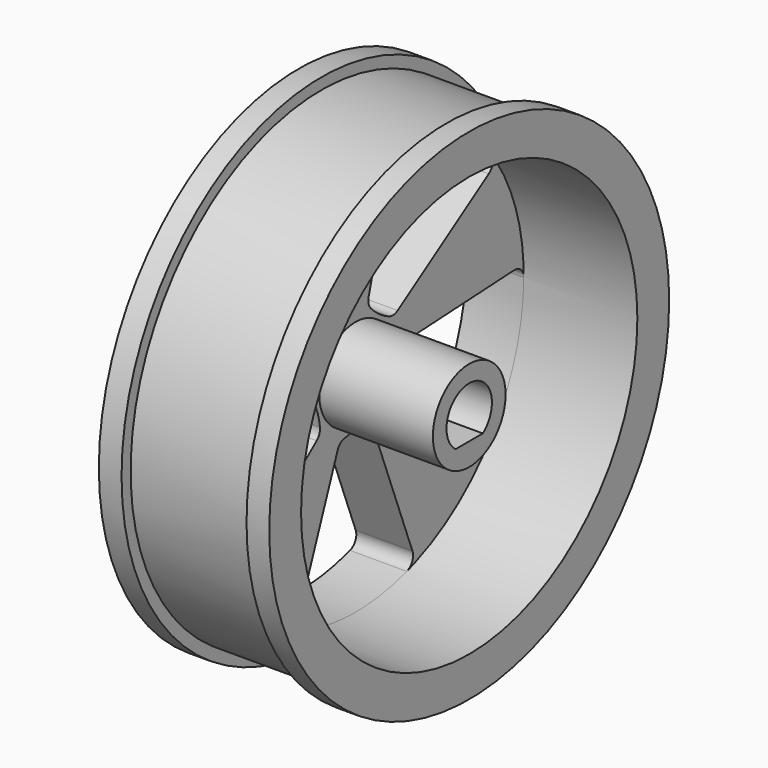
from build123d import *

# Parameters (mm, degrees)
F0_R         = 21
F1_DEPTH     = 5.5
F2_R         = 22
F3_DEPTH     = 2
F4_R         = 22
F5_DEPTH     = 2
F7_DEPTH     = 15.001
F8_R         = 18.5
F8_R_2       = 4
F9_DEPTH     = 10
F11_DEPTH    = 5.001
F12_T1_DEPTH = 5


# Not quite as in the source:
# - a fillet or chamfer that OpenCascade refuses, or shapes differently, is made with other operations: its cross-section is extruded or revolved along the edge and cut away or added


with BuildPart() as f1:
    # F0 (on Right) → F1 (new body, symmetric)
    with BuildSketch(Plane.YZ):
        Circle(F0_R)
    extrude(amount=F1_DEPTH, both=True)

    # F2 (on face) → F3 (join)
    with BuildSketch(Plane.YZ.offset(5.5)):
        Circle(F2_R)
    extrude(amount=F3_DEPTH)

    # F4 (on face) → F5 (join)
    with BuildSketch(Plane(origin=(-5.5, 0, 0), x_dir=(0, -1, 0), z_dir=(-1, 0, 0))):
        Circle(F4_R)
    extrude(amount=F5_DEPTH)

    # F6 (on face) → F7 (cut, through all)
    with BuildSketch(Plane(origin=(-7.5, 0, 0), x_dir=(0, -1, 0), z_dir=(-1, 0, 0))):
        with BuildLine():
            Line((-1.5, -2), (1.5, -2))
            ThreePointArc((1.5, -2), (0, 2.5), (-1.5, -2))
        make_face()
    extrude(amount=-F7_DEPTH, mode=Mode.SUBTRACT)

    # F8 (on face) → F9 (cut)
    with BuildSketch(Plane.YZ.offset(7.5)):
        Circle(F8_R)
        Circle(F8_R_2, mode=Mode.SUBTRACT)
    extrude(amount=-F9_DEPTH, mode=Mode.SUBTRACT)

    # F10 (on face) → F11 (cut, through all)
    with BuildSketch(Plane.YZ.offset(-2.5)):
        with BuildLine():
            Line((4.7881523344, 17.8696277863), (1.2940952255, 4.8296291314))
            ThreePointArc((1.2940952255, 4.8296291314), (2.5827855501, 3.5548993357), (4.1933528397, 2.7231951751))
            Line((4.1933528397, 2.7231951751), (15.515405507, 10.0758221478))
            ThreePointArc((15.515405507, 10.0758221478), (10.8740271674, 14.9668143959), (4.7881523344, 17.8696277863))
        make_face()
        with BuildLine():
            ThreePointArc((4.9931476738, 0.2616797812), (4.1790348058, -1.3578507196), (3.8857298073, -3.1466019552))
            Line((3.8857298073, -3.1466019552), (14.377200287, -11.6424272344))
            ThreePointArc((14.377200287, -11.6424272344), (17.5945455515, -5.7168143959), (18.474646393, 0.9682151905))
            Line((18.474646393, 0.9682151905), (4.9931476738, 0.2616797812))
        make_face()
        with BuildLine():
            ThreePointArc((1.7918397477, -4.6679021325), (0, -4.3940972321), (-1.7918397477, -4.6679021325))
            Line((-1.7918397477, -4.6679021325), (-6.6298070666, -17.2712378902))
            ThreePointArc((-6.6298070666, -17.2712378902), (0, -18.5), (6.6298070666, -17.2712378902))
            Line((6.6298070666, -17.2712378902), (1.7918397477, -4.6679021325))
        make_face()
        with BuildLine():
            ThreePointArc((-3.8857298073, -3.1466019552), (-4.1790348058, -1.3578507196), (-4.9931476738, 0.2616797812))
            Line((-4.9931476738, 0.2616797812), (-18.474646393, 0.9682151905))
            ThreePointArc((-18.474646393, 0.9682151905), (-17.5945455515, -5.7168143959), (-14.377200287, -11.6424272344))
            Line((-14.377200287, -11.6424272344), (-3.8857298073, -3.1466019552))
        make_face()
        with BuildLine():
            ThreePointArc((-4.1933528397, 2.7231951751), (-2.5827855501, 3.5548993357), (-1.2940952255, 4.8296291314))
            Line((-1.2940952255, 4.8296291314), (-4.7881523344, 17.8696277863))
            ThreePointArc((-4.7881523344, 17.8696277863), (-10.8740271674, 14.9668143959), (-15.515405507, 10.0758221478))
            Line((-15.515405507, 10.0758221478), (-4.1933528397, 2.7231951751))
        make_face()
    extrude(amount=-F11_DEPTH, mode=Mode.SUBTRACT)

    # F12: fillet of radius 1 on 20 edges, made by hand

    # F12_s2 → F12_t1 (join)
    with BuildSketch(Plane.YZ.offset(-7.5)):
        with BuildLine():
            ThreePointArc((4.6223226532, 3.0017714292), (4.1563467345, 2.8435407412), (3.671320929, 2.9267301361))
            ThreePointArc((3.671320929, 2.9267301361), (3.9299597122, 2.8188656209), (4.1933528397, 2.7231951751))
            Line((4.1933528397, 2.7231951751), (4.6223226532, 3.0017714292))
        make_face()
        with BuildLine():
            ThreePointArc((1.4264780248, 5.3236884645), (1.4199861758, 4.831623059), (1.6489852086, 4.3960430429))
            ThreePointArc((1.6489852086, 4.3960430429), (1.466476179, 4.6086911748), (1.2940952255, 4.8296291314))
            Line((1.2940952255, 4.8296291314), (1.4264780248, 5.3236884645))
        make_face()
        with BuildLine():
            ThreePointArc((14.65275333, 9.5156092737), (15.0918050058, 10.1744115971), (14.9142922547, 10.9459529755))
            ThreePointArc((14.9142922547, 10.9459529755), (15.221067912, 10.5151838604), (15.515405507, 10.0758221478))
            Line((15.515405507, 10.0758221478), (14.65275333, 9.5156092737))
        make_face()
        with BuildLine():
            ThreePointArc((4.521932413, 16.8760815136), (5.0128162263, 17.4972255847), (5.8014501386, 17.5668203238))
            ThreePointArc((5.8014501386, 17.5668203238), (5.2969654732, 17.7254663345), (4.7881523344, 17.8696277863))
            Line((4.7881523344, 17.8696277863), (4.521932413, 16.8760815136))
        make_face()
        with BuildLine():
            ThreePointArc((5.5039345567, 0.2884489874), (5.0339464546, 0.1425665301), (4.6904498348, -0.2098261196))
            ThreePointArc((4.6904498348, -0.2098261196), (4.8362918345, 0.0294621688), (4.9931476738, 0.2616797812))
            Line((4.9931476738, 0.2616797812), (5.5039345567, 0.2884489874))
        make_face()
        with BuildLine():
            ThreePointArc((4.2832305314, -3.4684916949), (3.9887497267, -3.0742182326), (3.9179863263, -2.5872243429))
            ThreePointArc((3.9179863263, -2.5872243429), (3.8953248556, -2.8665364113), (3.8857298073, -3.1466019552))
            Line((3.8857298073, -3.1466019552), (4.2832305314, -3.4684916949))
        make_face()
        with BuildLine():
            ThreePointArc((1.2498722119, -4.5257227166), (1.6911638308, -4.7435120977), (1.9751406031, -5.1454171863))
            Line((1.9751406031, -5.1454171863), (1.7918397477, -4.6679021325))
            ThreePointArc((1.7918397477, -4.6679021325), (1.5225165542, -4.5904825531), (1.2498722119, -4.5257227166))
        make_face()
        with BuildLine():
            ThreePointArc((-1.9751406031, -5.1454171863), (-1.6911638308, -4.7435120977), (-1.2498722119, -4.5257227166))
            ThreePointArc((-1.2498722119, -4.5257227166), (-1.5225165542, -4.5904825531), (-1.7918397477, -4.6679021325))
            Line((-1.7918397477, -4.6679021325), (-1.9751406031, -5.1454171863))
        make_face()
        with BuildLine():
            ThreePointArc((-5.5039345567, 0.2884489874), (-5.0339464546, 0.1425665301), (-4.6904498348, -0.2098261196))
            ThreePointArc((-4.6904498348, -0.2098261196), (-4.8362918345, 0.0294621688), (-4.9931476738, 0.2616797812))
            Line((-4.9931476738, 0.2616797812), (-5.5039345567, 0.2884489874))
        make_face()
        with BuildLine():
            ThreePointArc((-3.9179863263, -2.5872243429), (-3.9887497267, -3.0742182326), (-4.2832305314, -3.4684916949))
            Line((-4.2832305314, -3.4684916949), (-3.8857298073, -3.1466019552))
            ThreePointArc((-3.8857298073, -3.1466019552), (-3.8953248556, -2.8665364113), (-3.9179863263, -2.5872243429))
        make_face()
        with BuildLine():
            ThreePointArc((-3.671320929, 2.9267301361), (-4.1563467345, 2.8435407412), (-4.6223226532, 3.0017714292))
            Line((-4.6223226532, 3.0017714292), (-4.1933528397, 2.7231951751))
            ThreePointArc((-4.1933528397, 2.7231951751), (-3.9299597122, 2.8188656209), (-3.671320929, 2.9267301361))
        make_face()
        with BuildLine():
            ThreePointArc((-1.4264780248, 5.3236884645), (-1.4199861758, 4.831623059), (-1.6489852086, 4.3960430429))
            ThreePointArc((-1.6489852086, 4.3960430429), (-1.466476179, 4.6086911748), (-1.2940952255, 4.8296291314))
            Line((-1.2940952255, 4.8296291314), (-1.4264780248, 5.3236884645))
        make_face()
        with BuildLine():
            ThreePointArc((13.5778319997, -10.9951115587), (14.3400646715, -11.2090934022), (15.0189896702, -10.8018493457))
            ThreePointArc((15.0189896702, -10.8018493457), (14.7041027879, -11.2267253108), (14.377200287, -11.6424272344))
            Line((14.377200287, -11.6424272344), (13.5778319997, -10.9951115587))
        make_face()
        with BuildLine():
            ThreePointArc((17.447461256, 0.9143826986), (18.189895813, 0.639468523), (18.4997856244, -0.0890609411))
            ThreePointArc((18.4997856244, -0.0890609411), (18.4947726116, 0.4397568007), (18.474646393, 0.9682151905))
            Line((18.474646393, 0.9682151905), (17.447461256, 0.9143826986))
        make_face()
        with BuildLine():
            ThreePointArc((6.2611916607, -16.3109619271), (6.229157638, -17.1020123027), (5.6320461618, -17.6218630125))
            ThreePointArc((5.6320461618, -17.6218630125), (6.133432615, -17.4536816849), (6.6298070666, -17.2712378902))
            Line((6.6298070666, -17.2712378902), (6.2611916607, -16.3109619271))
        make_face()
        with BuildLine():
            ThreePointArc((-6.2611916607, -16.3109619271), (-6.229157638, -17.1020123027), (-5.6320461618, -17.6218630125))
            ThreePointArc((-5.6320461618, -17.6218630125), (-6.133432615, -17.4536816849), (-6.6298070666, -17.2712378902))
            Line((-6.6298070666, -17.2712378902), (-6.2611916607, -16.3109619271))
        make_face()
        with BuildLine():
            ThreePointArc((-17.447461256, 0.9143826986), (-18.189895813, 0.639468523), (-18.4997856244, -0.0890609411))
            ThreePointArc((-18.4997856244, -0.0890609411), (-18.4947726116, 0.4397568007), (-18.474646393, 0.9682151905))
            Line((-18.474646393, 0.9682151905), (-17.447461256, 0.9143826986))
        make_face()
        with BuildLine():
            ThreePointArc((-13.5778319997, -10.9951115587), (-14.3400646715, -11.2090934022), (-15.0189896702, -10.8018493457))
            ThreePointArc((-15.0189896702, -10.8018493457), (-14.7041027879, -11.2267253108), (-14.377200287, -11.6424272344))
            Line((-14.377200287, -11.6424272344), (-13.5778319997, -10.9951115587))
        make_face()
        with BuildLine():
            ThreePointArc((-4.521932413, 16.8760815136), (-5.0128162263, 17.4972255847), (-5.8014501386, 17.5668203238))
            ThreePointArc((-5.8014501386, 17.5668203238), (-5.2969654732, 17.7254663345), (-4.7881523344, 17.8696277863))
            Line((-4.7881523344, 17.8696277863), (-4.521932413, 16.8760815136))
        make_face()
        with BuildLine():
            ThreePointArc((-14.65275333, 9.5156092737), (-15.0918050058, 10.1744115971), (-14.9142922547, 10.9459529755))
            ThreePointArc((-14.9142922547, 10.9459529755), (-15.221067912, 10.5151838604), (-15.515405507, 10.0758221478))
            Line((-15.515405507, 10.0758221478), (-14.65275333, 9.5156092737))
        make_face()
    extrude(amount=F12_T1_DEPTH)


solid = f1.part
